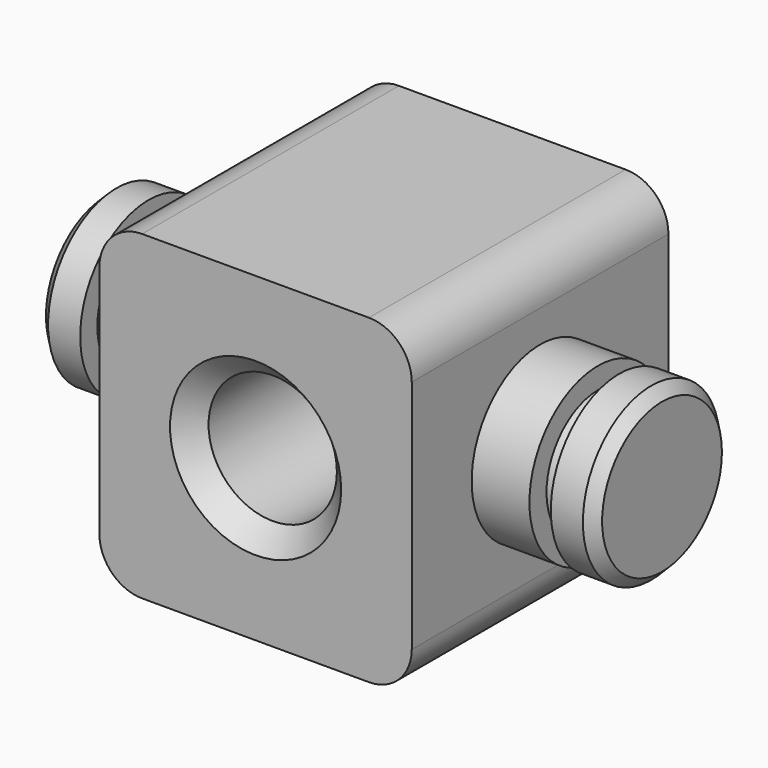
from build123d import *

# Parameters (mm, degrees)
F0_W     = 14.6
F0_H     = 15
F0_R     = 3
F1_DEPTH = 7.5
F2_SIZE  = 1
F3_R     = 4
F4_DEPTH = 5.7
F5_W     = 1
F5_H     = 1
F7_SIZE  = 0.5
F8_R     = 2


# Not quite as in the source:
# - a pattern or mirror of a feature is missing from the dataset's text; its kind, count and spacing are read off the source's solid


with BuildPart() as f1:
    # F0 (on Front) → F1 (new body, symmetric)
    with BuildSketch(Plane.XZ):
        Rectangle(F0_W, F0_H)
        Circle(F0_R, mode=Mode.SUBTRACT)
    extrude(amount=F1_DEPTH, both=True)

    # F2
    f2_edges = [f1.edges().sort_by_distance(p)[0] for p in [
        (-3, -7.5, 0),
        (-3, 7.5, 0),
    ]]
    chamfer(f2_edges, length=F2_SIZE)

    # F3 (on face) → F4 (join)
    with BuildSketch(Plane.YZ.offset(7.3)):
        Circle(F3_R)
    f4 = extrude(amount=F4_DEPTH)

    # F4_copies: F4 across plane
    add(f4.mirror(Plane(origin=(0, 0, 0), x_dir=(0, 0, -1), z_dir=(-1, 0, 0))))

    # F5 (on Front) → F6 (revolve, cut)
    with BuildSketch(Plane.XZ):
        with Locations((10.5, 3.5)):
            Rectangle(F5_W, F5_H)
    f6 = revolve(axis=Axis((10.5, 0, 0), (-1, 0, 0)), mode=Mode.SUBTRACT)

    # F6_copies: F6 across plane
    add(f6.mirror(Plane(origin=(0, 0, 0), x_dir=(0, 0, -1), z_dir=(-1, 0, 0))), mode=Mode.SUBTRACT)

    # F7
    f7_edges = [f1.edges().sort_by_distance(p)[0] for p in [
        (13, -4, 0),
        (-13, -4, 0),
    ]]
    chamfer(f7_edges, length=F7_SIZE)

    # F8
    f8_edges = [f1.edges().sort_by_distance(p)[0] for p in [
        (-7.3, 0, 7.5),
        (7.3, 0, 7.5),
        (-7.3, 0, -7.5),
        (7.3, 0, -7.5),
    ]]
    fillet(f8_edges, radius=F8_R)


solid = f1.part
